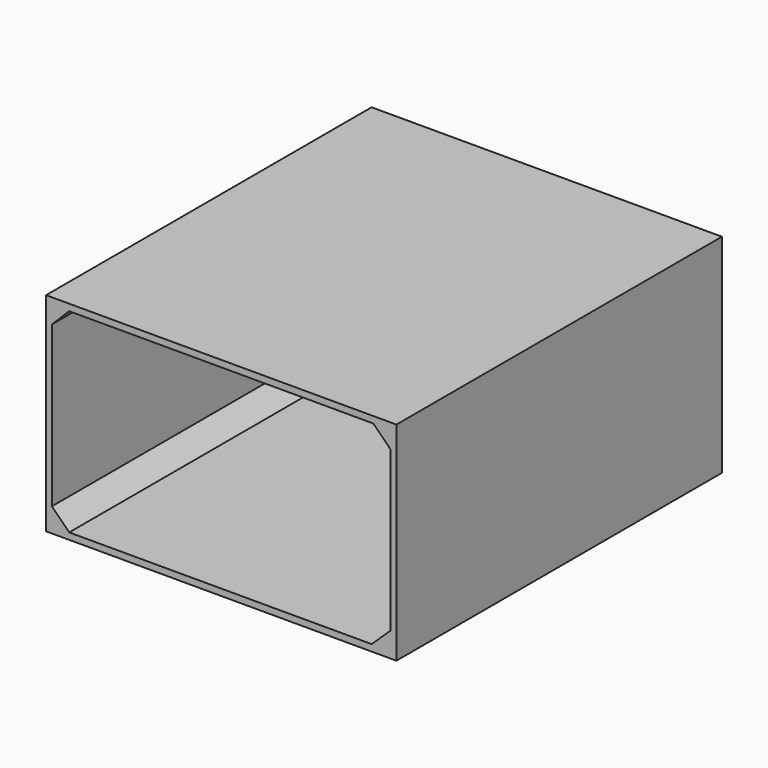
from build123d import *

# Parameters (mm, degrees)
F0_W     = 460.375
F0_H     = 534.67
F1_DEPTH = 273.2278
F3_DEPTH = 536.956


# Not quite as in the source:
# - a feature names something its author has since deleted; it is built from what else it names


with BuildPart() as f1:
    # F0 (on Top) → F1 (new body)
    with BuildSketch(Plane.XY):
        with Locations((230.1875, 267.335)):
            Rectangle(F0_W, F0_H)
    extrude(amount=F1_DEPTH)

    # F2 (on face) → F3 (cut)
    with BuildSketch(Plane.XZ):
        Polygon((452.7307115978, 241.8399496412), (430.0117425975, 264.584589793), (30.3632574025, 264.584589793), (7.6442884022, 241.8399496412), (7.6442884022, 31.3878503588), (30.3632574025, 8.643210207), (427.9011, 8.643210207), (452.7307115978, 32.4993), align=None)
    extrude(amount=-F3_DEPTH, mode=Mode.SUBTRACT)


solid = f1.part
